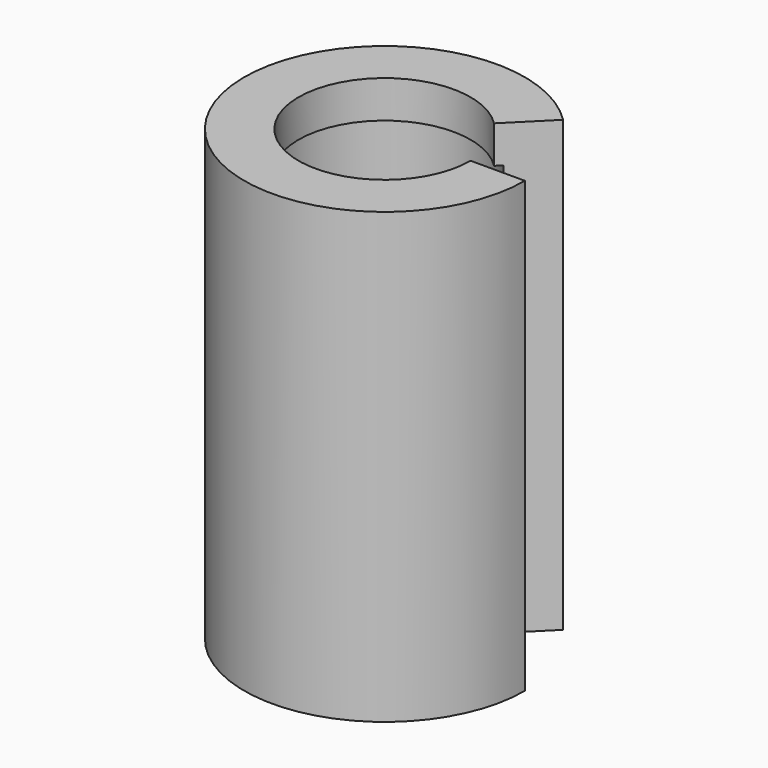
from build123d import *

# Parameters (mm, degrees)
F1_DEPTH = 2
F3_DEPTH = 20
F5_DEPTH = 2


with BuildPart() as f1:
    # F0 (on Top) → F1 (new body)
    with BuildSketch(Plane.XY):
        with BuildLine():
            ThreePointArc((5.3033008589, 5.3033008589), (-6.9290964938, -2.8701257427), (7.5, 0))
            Line((7.5, 0), (5, 0))
            ThreePointArc((5, 0), (-4.6193976626, -1.9134171618), (3.5355339059, 3.5355339059))
            Line((3.5355339059, 3.5355339059), (5.3033008589, 5.3033008589))
        make_face()
        with BuildLine():
            ThreePointArc((3.5355339059, 3.5355339059), (-4.6193976626, -1.9134171618), (5, 0))
            Line((5, 0), (4.6, 0))
            ThreePointArc((4.6, 0), (-4.2498458496, -1.7603437889), (3.2526911935, 3.2526911935))
            Line((3.2526911935, 3.2526911935), (3.5355339059, 3.5355339059))
        make_face()
    extrude(amount=F1_DEPTH)

    # F2 (on face) → F3 (join)
    with BuildSketch(Plane.XY.offset(2)):
        with BuildLine():
            Line((7.5, 0), (5, 0))
            ThreePointArc((5, 0), (-4.6193976626, -1.9134171618), (3.5355339059, 3.5355339059))
            Line((3.5355339059, 3.5355339059), (5.3033008589, 5.3033008589))
            ThreePointArc((5.3033008589, 5.3033008589), (-6.9290964938, -2.8701257427), (7.5, 0))
        make_face()
    extrude(amount=F3_DEPTH)

    # F4 (on face) → F5 (join)
    with BuildSketch(Plane.XY.offset(22)):
        with BuildLine():
            ThreePointArc((3.5355339059, 3.5355339059), (-4.6193976626, -1.9134171618), (5, 0))
            Line((5, 0), (4.6, 0))
            ThreePointArc((4.6, 0), (-4.2498458496, -1.7603437889), (3.2526911935, 3.2526911935))
            Line((3.2526911935, 3.2526911935), (3.5355339059, 3.5355339059))
        make_face()
        with BuildLine():
            ThreePointArc((5.3033008589, 5.3033008589), (-6.9290964938, -2.8701257427), (7.5, 0))
            Line((7.5, 0), (5, 0))
            ThreePointArc((5, 0), (-4.6193976626, -1.9134171618), (3.5355339059, 3.5355339059))
            Line((3.5355339059, 3.5355339059), (5.3033008589, 5.3033008589))
        make_face()
    extrude(amount=F5_DEPTH)


solid = f1.part
